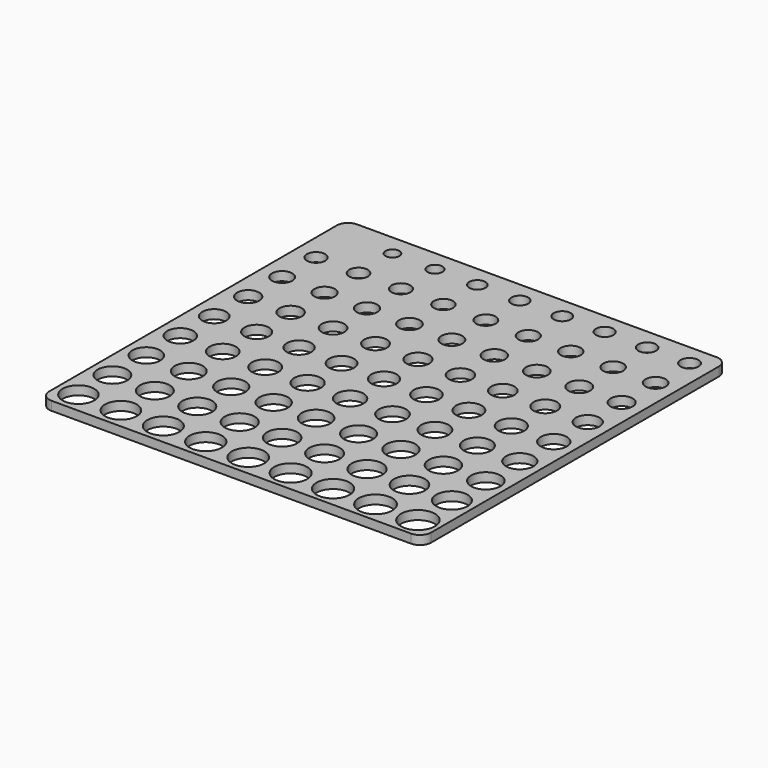
from build123d import *

# Parameters (mm, degrees)
F1_W     = 272.43
F1_H     = 272.43
F2_DEPTH = 6.35
F3_D     = 9.91
F4_D     = 10.72
F5_D     = 11.53
F6_D     = 11.95
F7_D     = 12.18
F8_D     = 12.37
F9_D     = 12.6
F10_D    = 12.78
F11_D    = 13
F12_D    = 13.21
F13_D    = 13.41
F14_D    = 13.61
F15_D    = 13.83
F16_D    = 14.05
F17_D    = 14.15
F18_D    = 14.25
F19_D    = 14.36
F20_D    = 14.45
F21_D    = 14.56
F22_D    = 14.65
F23_D    = 14.86
F24_D    = 15.04
F25_D    = 15.27
F26_D    = 15.4
F27_D    = 15.53
F28_D    = 15.7
F29_D    = 15.8
F30_D    = 15.9
F31_D    = 16
F32_D    = 16.1
F33_D    = 16.3
F34_D    = 16.41
F35_D    = 16.51
F36_D    = 16.71
F37_D    = 16.92
F38_D    = 17.13
F39_D    = 17.35
F40_R    = 8
F41_D    = 17.45
F42_D    = 17.75
F43_D    = 17.97
F44_D    = 18.19
F45_D    = 18.35
F46_D    = 18.53
F47_D    = 18.61
F48_D    = 18.69
F49_D    = 18.8
F50_D    = 18.89
F51_D    = 19.1
F52_D    = 19.22
F53_D    = 19.31
F54_D    = 19.41
F55_D    = 19.51
F56_D    = 19.62
F57_D    = 19.84
F58_D    = 20.02
F59_D    = 20.2
F60_D    = 20.32
F61_D    = 20.44
F62_D    = 20.68
F63_D    = 20.76
F64_D    = 20.85
F65_D    = 20.94
F66_D    = 21.08
F67_D    = 21.18
F68_D    = 21.24
F69_D    = 21.3
F70_D    = 21.49
F71_D    = 21.69
F72_D    = 21.89
F73_D    = 22.1
F74_D    = 22.33
F75_D    = 22.6
F76_D    = 22.69
F77_D    = 22.92
F78_D    = 23.06
F79_D    = 23.24
F80_D    = 23.47
F81_D    = 23.55
F82_D    = 23.87
F83_D    = 24.27


# Not quite as in the source:
# - a length typed as a fraction of an inch, garbled in the dataset ("3 / 203.2 mm" for 3/8 in), is restored


with BuildPart() as f2:
    # F1 (on Top) → F2 (new body)
    with BuildSketch(Plane.XY):
        with Locations((136.215, -136.215)):
            Rectangle(F1_W, F1_H)
    extrude(amount=-F2_DEPTH)

    # F3 (through all)
    with Locations(Plane.XY):
        with Locations((45.405, -15.135)):
            Hole(F3_D / 2)

    # F4 (through all)
    with Locations(Plane.XY):
        with Locations((75.675, -15.135)):
            Hole(F4_D / 2)

    # F5 (through all)
    with Locations(Plane.XY):
        with Locations((105.945, -15.135)):
            Hole(F5_D / 2)

    # F6 (through all)
    with Locations(Plane.XY):
        with Locations((136.215, -15.135)):
            Hole(F6_D / 2)

    # F7 (through all)
    with Locations(Plane.XY):
        with Locations((166.485, -15.135)):
            Hole(F7_D / 2)

    # F8 (through all)
    with Locations(Plane.XY):
        with Locations((196.755, -15.135)):
            Hole(F8_D / 2)

    # F9 (through all)
    with Locations(Plane.XY):
        with Locations((227.025, -15.135)):
            Hole(F9_D / 2)

    # F10 (through all)
    with Locations(Plane.XY):
        with Locations((257.295, -15.135)):
            Hole(F10_D / 2)

    # F11 (through all)
    with Locations(Plane.XY):
        with Locations((15.135, -45.405)):
            Hole(F11_D / 2)

    # F12 (through all)
    with Locations(Plane.XY):
        with Locations((45.405, -45.405)):
            Hole(F12_D / 2)

    # F13 (through all)
    with Locations(Plane.XY):
        with Locations((75.675, -45.405)):
            Hole(F13_D / 2)

    # F14 (through all)
    with Locations(Plane.XY):
        with Locations((105.945, -45.405)):
            Hole(F14_D / 2)

    # F15 (through all)
    with Locations(Plane.XY):
        with Locations((136.215, -45.405)):
            Hole(F15_D / 2)

    # F16 (through all)
    with Locations(Plane.XY):
        with Locations((166.485, -45.405)):
            Hole(F16_D / 2)

    # F17 (through all)
    with Locations(Plane.XY):
        with Locations((196.755, -45.405)):
            Hole(F17_D / 2)

    # F18 (through all)
    with Locations(Plane.XY):
        with Locations((227.025, -45.405)):
            Hole(F18_D / 2)

    # F19 (through all)
    with Locations(Plane.XY):
        with Locations((257.295, -45.405)):
            Hole(F19_D / 2)

    # F20 (through all)
    with Locations(Plane.XY):
        with Locations((15.135, -75.675)):
            Hole(F20_D / 2)

    # F21 (through all)
    with Locations(Plane.XY):
        with Locations((45.405, -75.675)):
            Hole(F21_D / 2)

    # F22 (through all)
    with Locations(Plane.XY):
        with Locations((75.675, -75.675)):
            Hole(F22_D / 2)

    # F23 (through all)
    with Locations(Plane.XY):
        with Locations((105.945, -75.675)):
            Hole(F23_D / 2)

    # F24 (through all)
    with Locations(Plane.XY):
        with Locations((136.215, -75.675)):
            Hole(F24_D / 2)

    # F25 (through all)
    with Locations(Plane.XY):
        with Locations((166.485, -75.675)):
            Hole(F25_D / 2)

    # F26 (through all)
    with Locations(Plane.XY):
        with Locations((196.755, -75.675)):
            Hole(F26_D / 2)

    # F27 (through all)
    with Locations(Plane.XY):
        with Locations((227.025, -75.675)):
            Hole(F27_D / 2)

    # F28 (through all)
    with Locations(Plane.XY):
        with Locations((257.295, -75.675)):
            Hole(F28_D / 2)

    # F29 (through all)
    with Locations(Plane.XY):
        with Locations((15.135, -105.945)):
            Hole(F29_D / 2)

    # F30 (through all)
    with Locations(Plane.XY):
        with Locations((45.405, -105.945)):
            Hole(F30_D / 2)

    # F31 (through all)
    with Locations(Plane.XY):
        with Locations((75.675, -105.945)):
            Hole(F31_D / 2)

    # F32 (through all)
    with Locations(Plane.XY):
        with Locations((105.945, -105.945)):
            Hole(F32_D / 2)

    # F33 (through all)
    with Locations(Plane.XY):
        with Locations((136.215, -105.945)):
            Hole(F33_D / 2)

    # F34 (through all)
    with Locations(Plane.XY):
        with Locations((166.485, -105.945)):
            Hole(F34_D / 2)

    # F35 (through all)
    with Locations(Plane.XY):
        with Locations((196.755, -105.945)):
            Hole(F35_D / 2)

    # F36 (through all)
    with Locations(Plane.XY):
        with Locations((227.025, -105.945)):
            Hole(F36_D / 2)

    # F37 (through all)
    with Locations(Plane.XY):
        with Locations((257.295, -105.945)):
            Hole(F37_D / 2)

    # F38 (through all)
    with Locations(Plane.XY):
        with Locations((15.135, -136.215)):
            Hole(F38_D / 2)

    # F39 (through all)
    with Locations(Plane.XY):
        with Locations((45.405, -136.215)):
            Hole(F39_D / 2)

    # F40
    f40_edges = [f2.edges().sort_by_distance(p)[0] for p in [
        (0, 0, -3.175),
        (272.43, 0, -3.175),
        (272.43, -272.43, -3.175),
        (0, -272.43, -3.175),
    ]]
    fillet(f40_edges, radius=F40_R)

    # F41 (through all)
    with Locations(Plane.XY):
        with Locations((75.675, -136.215)):
            Hole(F41_D / 2)

    # F42 (through all)
    with Locations(Plane.XY):
        with Locations((105.945, -136.215)):
            Hole(F42_D / 2)

    # F43 (through all)
    with Locations(Plane.XY):
        with Locations((136.215, -136.215)):
            Hole(F43_D / 2)

    # F44 (through all)
    with Locations(Plane.XY):
        with Locations((166.485, -136.215)):
            Hole(F44_D / 2)

    # F45 (through all)
    with Locations(Plane.XY):
        with Locations((196.755, -136.215)):
            Hole(F45_D / 2)

    # F46 (through all)
    with Locations(Plane.XY):
        with Locations((227.025, -136.215)):
            Hole(F46_D / 2)

    # F47 (through all)
    with Locations(Plane.XY):
        with Locations((257.295, -136.215)):
            Hole(F47_D / 2)

    # F48 (through all)
    with Locations(Plane.XY):
        with Locations((15.135, -166.485)):
            Hole(F48_D / 2)

    # F49 (through all)
    with Locations(Plane.XY):
        with Locations((45.405, -166.485)):
            Hole(F49_D / 2)

    # F50 (through all)
    with Locations(Plane.XY):
        with Locations((75.675, -166.485)):
            Hole(F50_D / 2)

    # F51 (through all)
    with Locations(Plane.XY):
        with Locations((105.945, -166.485)):
            Hole(F51_D / 2)

    # F52 (through all)
    with Locations(Plane.XY):
        with Locations((136.215, -166.485)):
            Hole(F52_D / 2)

    # F53 (through all)
    with Locations(Plane.XY):
        with Locations((166.485, -166.485)):
            Hole(F53_D / 2)

    # F54 (through all)
    with Locations(Plane.XY):
        with Locations((196.755, -166.485)):
            Hole(F54_D / 2)

    # F55 (through all)
    with Locations(Plane.XY):
        with Locations((227.025, -166.485)):
            Hole(F55_D / 2)

    # F56 (through all)
    with Locations(Plane.XY):
        with Locations((257.295, -166.485)):
            Hole(F56_D / 2)

    # F57 (through all)
    with Locations(Plane.XY):
        with Locations((15.135, -196.755)):
            Hole(F57_D / 2)

    # F58 (through all)
    with Locations(Plane.XY):
        with Locations((45.405, -196.755)):
            Hole(F58_D / 2)

    # F59 (through all)
    with Locations(Plane.XY):
        with Locations((75.675, -196.755)):
            Hole(F59_D / 2)

    # F60 (through all)
    with Locations(Plane.XY):
        with Locations((105.945, -196.755)):
            Hole(F60_D / 2)

    # F61 (through all)
    with Locations(Plane.XY):
        with Locations((136.215, -196.755)):
            Hole(F61_D / 2)

    # F62 (through all)
    with Locations(Plane.XY):
        with Locations((166.485, -196.755)):
            Hole(F62_D / 2)

    # F63 (through all)
    with Locations(Plane.XY):
        with Locations((196.755, -196.755)):
            Hole(F63_D / 2)

    # F64 (through all)
    with Locations(Plane.XY):
        with Locations((227.025, -196.755)):
            Hole(F64_D / 2)

    # F65 (through all)
    with Locations(Plane.XY):
        with Locations((257.295, -196.755)):
            Hole(F65_D / 2)

    # F66 (through all)
    with Locations(Plane.XY):
        with Locations((15.135, -227.025)):
            Hole(F66_D / 2)

    # F67 (through all)
    with Locations(Plane.XY):
        with Locations((45.405, -227.025)):
            Hole(F67_D / 2)

    # F68 (through all)
    with Locations(Plane.XY):
        with Locations((75.675, -227.025)):
            Hole(F68_D / 2)

    # F69 (through all)
    with Locations(Plane.XY):
        with Locations((105.945, -227.025)):
            Hole(F69_D / 2)

    # F70 (through all)
    with Locations(Plane.XY):
        with Locations((136.215, -227.025)):
            Hole(F70_D / 2)

    # F71 (through all)
    with Locations(Plane.XY):
        with Locations((166.485, -227.025)):
            Hole(F71_D / 2)

    # F72 (through all)
    with Locations(Plane.XY):
        with Locations((196.755, -227.025)):
            Hole(F72_D / 2)

    # F73 (through all)
    with Locations(Plane.XY):
        with Locations((227.025, -227.025)):
            Hole(F73_D / 2)

    # F74 (through all)
    with Locations(Plane.XY):
        with Locations((257.295, -227.025)):
            Hole(F74_D / 2)

    # F75 (through all)
    with Locations(Plane.XY):
        with Locations((15.135, -257.295)):
            Hole(F75_D / 2)

    # F76 (through all)
    with Locations(Plane.XY):
        with Locations((45.405, -257.295)):
            Hole(F76_D / 2)

    # F77 (through all)
    with Locations(Plane.XY):
        with Locations((75.675, -257.295)):
            Hole(F77_D / 2)

    # F78 (through all)
    with Locations(Plane.XY):
        with Locations((105.945, -257.295)):
            Hole(F78_D / 2)

    # F79 (through all)
    with Locations(Plane.XY):
        with Locations((136.215, -257.295)):
            Hole(F79_D / 2)

    # F80 (through all)
    with Locations(Plane.XY):
        with Locations((166.485, -257.295)):
            Hole(F80_D / 2)

    # F81 (through all)
    with Locations(Plane.XY):
        with Locations((196.755, -257.295)):
            Hole(F81_D / 2)

    # F82 (through all)
    with Locations(Plane.XY):
        with Locations((227.025, -257.295)):
            Hole(F82_D / 2)

    # F83 (through all)
    with Locations(Plane.XY):
        with Locations((257.295, -257.295)):
            Hole(F83_D / 2)


solid = f2.part
